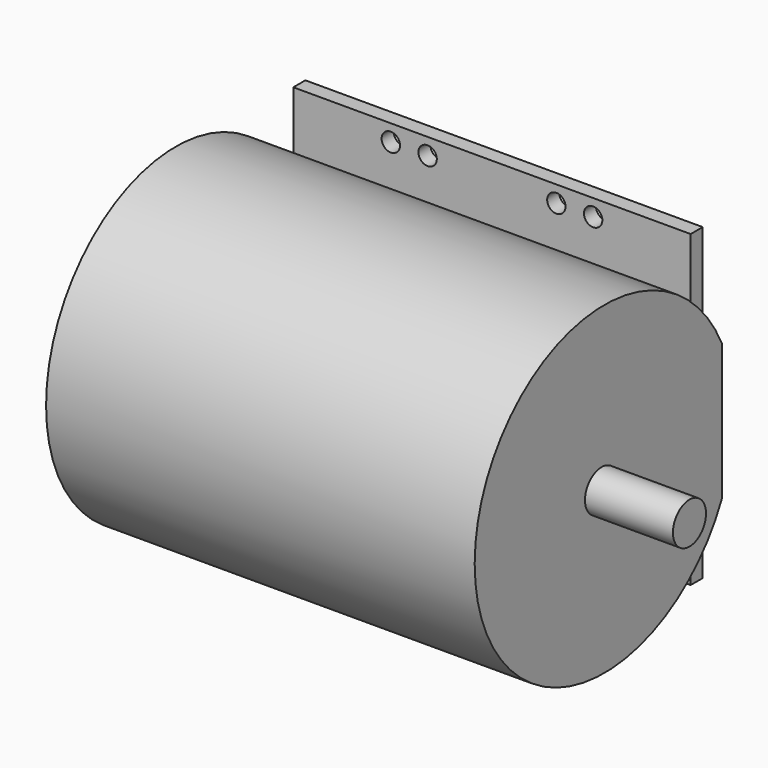
from build123d import *

# Parameters (mm, degrees)
F0_W          = 274.32
F0_H          = 213.36
F0_R          = 6.35
F1_DEPTH      = 10.414
F3_DEPTH      = 21.59
F3_DEPTH_BACK = 274.32
F4_R          = 14.2875
F5_DEPTH      = 60.706


with BuildPart() as f1:
    # F0 (on Front) → F1 (new body)
    with BuildSketch(Plane.XZ):
        with Locations((-81.1550752527, 15.3063097969)):
            Rectangle(F0_W, F0_H)
        with Locations((-151.0050752527, -79.9436902031)):
            Circle(F0_R, mode=Mode.SUBTRACT)
        with Locations((-125.6050752527, -79.9436902031)):
            Circle(F0_R, mode=Mode.SUBTRACT)
        with Locations((-36.7050752527, -79.9436902031)):
            Circle(F0_R, mode=Mode.SUBTRACT)
        with Locations((-11.3050752527, -79.9436902031)):
            Circle(F0_R, mode=Mode.SUBTRACT)
        with Locations((-151.0050752527, 110.5563097969)):
            Circle(F0_R, mode=Mode.SUBTRACT)
        with Locations((-125.6050752527, 110.5563097969)):
            Circle(F0_R, mode=Mode.SUBTRACT)
        with Locations((-36.7050752527, 110.5563097969)):
            Circle(F0_R, mode=Mode.SUBTRACT)
        with Locations((-11.3050752527, 110.5563097969)):
            Circle(F0_R, mode=Mode.SUBTRACT)
    extrude(amount=F1_DEPTH)

    # F2 (on face) → F3 (join, two sides)
    with BuildSketch(Plane.YZ.offset(56.0049247473)) as f3_sk:
        with BuildLine():
            Line((-10.414, -31.8310537272), (-10.414, 62.4436733209))
            ThreePointArc((-10.414, 62.4436733209), (-223.774, 15.3063097969), (-10.414, -31.8310537272))
        make_face()
    extrude(amount=F3_DEPTH)
    extrude(f3_sk.sketch, amount=-F3_DEPTH_BACK)

    # F4 (on face) → F5 (join)
    with BuildSketch(Plane.YZ.offset(77.5949247473)):
        with Locations((-114.3, 15.3063097969)):
            Circle(F4_R)
    extrude(amount=F5_DEPTH)


solid = f1.part
